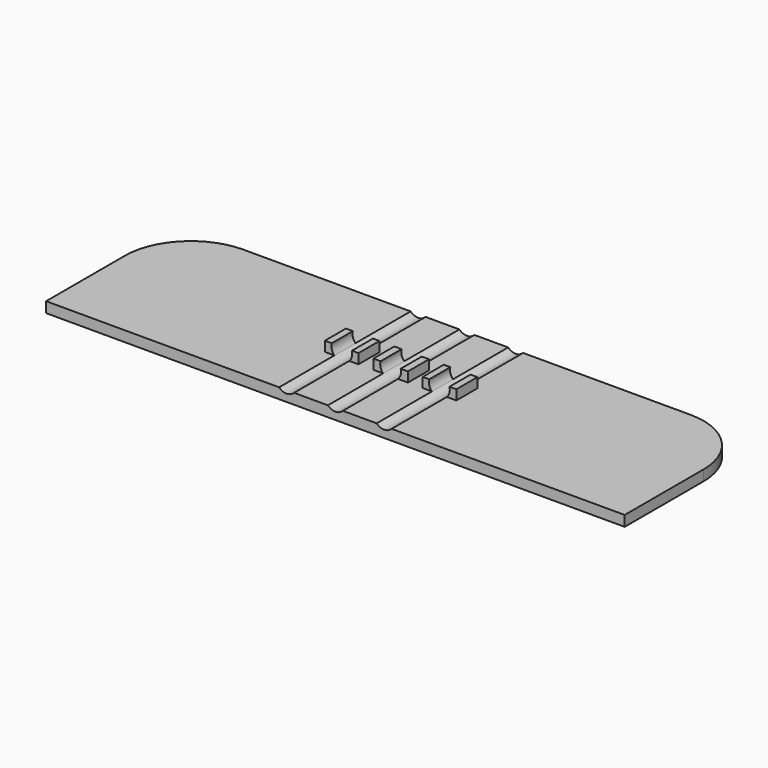
from build123d import *

# Parameters (mm, degrees)
F0_W        = 152.4
F0_H        = 76.2
F1_DEPTH    = 10.16
F3_DEPTH    = 254
F4_W        = 114.3
F4_H        = 76.2
F5_DEPTH    = 5.08
F6_T1_DEPTH = 120.65
F6_T6_DEPTH = 120.65
F8_W        = 223.52
F8_H        = 63.5
F9_DEPTH    = 2.794
F10_W       = 50.8
F10_H       = 10.16
F11_DEPTH   = 3.81
F13_DEPTH   = 63.5
F14_W       = 5.715
F14_H       = 3.81
F15_DEPTH   = 25.4
F16_R       = 25.4
F17_DEPTH   = 1.27


# Not quite as in the source:
# - a fillet or chamfer that OpenCascade refuses, or shapes differently, is made with other operations: its cross-section is extruded or revolved along the edge and cut away or added


with BuildPart() as f1:
    # F0 (on Top) → F1 (new body)
    with BuildSketch(Plane.XY):
        Rectangle(F0_W, F0_H)
    extrude(amount=F1_DEPTH)

    # F2 (on face) → F3 (cut)
    with BuildSketch(Plane.XZ.offset(38.1)):
        with BuildLine():
            ThreePointArc((-71.670055, 10.16), (-69.929038, 3.854348), (-64.579995, 7.62))
            ThreePointArc((-64.579995, 7.62), (-64.814348, 8.969038), (-65.489945, 10.16))
            Line((-65.489945, 10.16), (-71.670055, 10.16))
        make_face()
        with BuildLine():
            Line((-49.487945, 10.16), (-55.668055, 10.16))
            ThreePointArc((-55.668055, 10.16), (-53.927038, 3.854348), (-48.577995, 7.62))
            ThreePointArc((-48.577995, 7.62), (-48.812348, 8.969038), (-49.487945, 10.16))
        make_face()
    extrude(amount=-F3_DEPTH, mode=Mode.SUBTRACT)

    # F4 (on face) → F5 (cut)
    with BuildSketch(Plane(origin=(0, 0, 0), x_dir=(1, 0, 0), z_dir=(0, 0, -1))):
        with Locations((19.05, 0)):
            Rectangle(F4_W, F4_H)
    extrude(amount=-F5_DEPTH, mode=Mode.SUBTRACT)

    # F6: fillet of radius 8.89 on 2 edges, made by hand

    # F6_s2 → F6_t1 (cut)
    with BuildSketch(Plane.XZ.offset(-60.325)):
        with BuildLine():
            ThreePointArc((-67.31, 0), (-73.596179, 2.603821), (-76.2, 8.89))
            Line((-76.2, 8.89), (-76.2, 0))
            Line((-76.2, 0), (-67.31, 0))
        make_face()
    extrude(amount=F6_T1_DEPTH, mode=Mode.SUBTRACT)


with BuildPart() as f6_tool4:
    # F6_s5 → F6_t6 (new body)
    with BuildSketch(Plane.XZ.offset(60.325)):
        with BuildLine():
            ThreePointArc((-46.99, 0), (-40.703821, 2.603821), (-38.1, 8.89))
            Line((-38.1, 8.89), (-38.1, 0))
            Line((-38.1, 0), (-46.99, 0))
        make_face()
    extrude(amount=-F6_T6_DEPTH)

    split(bisect_by=Plane.XY.offset(5.08), keep=Keep.BOTTOM)


with BuildPart() as f1_1:
    add(f1.part)

    # F6_t3: cut F6_tool4
    add(f6_tool4.part, mode=Mode.SUBTRACT)


with BuildPart() as f9:
    # F8 (on Top) → F9 (new body)
    with BuildSketch(Plane.XY):
        Rectangle(F8_W, F8_H)
    extrude(amount=F9_DEPTH)

    # F10 (on face) → F11 (join)
    with BuildSketch(Plane.XY.offset(2.794)):
        Rectangle(F10_W, F10_H)
    extrude(amount=F11_DEPTH)

    # F12 (on face) → F13 (cut, symmetric)
    with BuildSketch(Plane.XZ.offset(5.08)):
        with BuildLine():
            ThreePointArc((2.889697, 2.794), (3.726397, 4.081099), (4.01955, 5.588))
            ThreePointArc((4.01955, 5.588), (3.986786, 6.100175), (3.889026, 6.604))
            Line((3.889026, 6.604), (-3.889026, 6.604))
            ThreePointArc((-3.889026, 6.604), (-3.888032, 4.568203), (-2.889697, 2.794))
            Line((-2.889697, 2.794), (2.889697, 2.794))
        make_face()
        with BuildLine():
            Line((22.729476, 6.604), (14.951424, 6.604))
            ThreePointArc((14.951424, 6.604), (14.952418, 4.568203), (15.950753, 2.794))
            Line((15.950753, 2.794), (21.730147, 2.794))
            ThreePointArc((21.730147, 2.794), (22.566847, 4.081099), (22.86, 5.588))
            ThreePointArc((22.86, 5.588), (22.827236, 6.100175), (22.729476, 6.604))
        make_face()
        with BuildLine():
            ThreePointArc((-2.889697, 2.794), (0, 1.56845), (2.889697, 2.794))
            Line((2.889697, 2.794), (-2.889697, 2.794))
        make_face()
        with BuildLine():
            Line((21.730147, 2.794), (15.950753, 2.794))
            ThreePointArc((15.950753, 2.794), (18.84045, 1.56845), (21.730147, 2.794))
        make_face()
        with BuildLine():
            ThreePointArc((-14.8209, 5.588), (-14.853664, 6.100175), (-14.951424, 6.604))
            Line((-14.951424, 6.604), (-22.729476, 6.604))
            ThreePointArc((-22.729476, 6.604), (-22.728482, 4.568203), (-21.730147, 2.794))
            Line((-21.730147, 2.794), (-15.950753, 2.794))
            ThreePointArc((-15.950753, 2.794), (-15.114053, 4.081099), (-14.8209, 5.588))
        make_face()
        with BuildLine():
            ThreePointArc((-21.730147, 2.794), (-18.84045, 1.56845), (-15.950753, 2.794))
            Line((-15.950753, 2.794), (-21.730147, 2.794))
        make_face()
    extrude(amount=F13_DEPTH, both=True, mode=Mode.SUBTRACT)

    # F14 (on face) → F15 (cut)
    with BuildSketch(Plane.XZ.offset(5.08)):
        with Locations((-9.554918, 4.699)):
            Rectangle(F14_W, F14_H)
        with Locations((9.554918, 4.699)):
            Rectangle(F14_W, F14_H)
    extrude(amount=-F15_DEPTH, mode=Mode.SUBTRACT)

    # F16
    f16_edges = [f9.edges().sort_by_distance(p)[0] for p in [
        (111.76, 31.75, 1.397),
        (-111.76, 31.75, 1.397),
    ]]
    fillet(f16_edges, radius=F16_R)

    # F17 (add): a face of the model
    f17_faces = [f9.faces().sort_by_distance(p)[0] for p in [
        (0, -0.518855, 0),
    ]]
    extrude(f17_faces, amount=F17_DEPTH)


solid = f9.part
